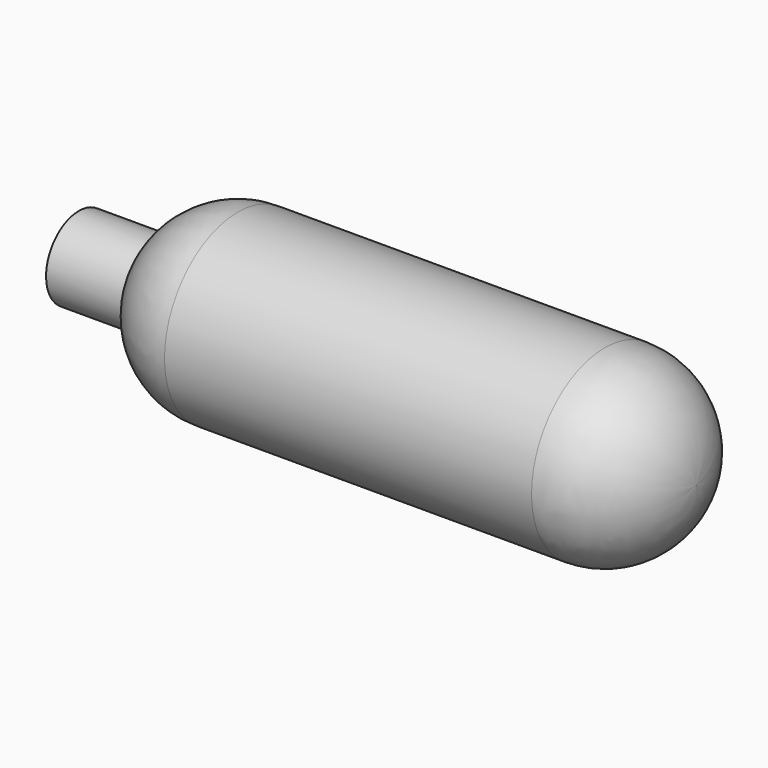
from build123d import *


# Not quite as in the source:
# - a fillet or chamfer that OpenCascade refuses, or shapes differently, is made with other operations: its cross-section is extruded or revolved along the edge and cut away or added


with BuildPart() as f1:
    # F0 (on Front) → F1 (revolve)
    with BuildSketch(Plane.XZ):
        Polygon((0, 4.2418), (0, 0), (64.008, 0), (64.008, 9.4996), (56.007, 9.4996), (36.0045, 9.4996), (16.002, 9.4996), (8.001, 9.4996), (8.001, 4.2418), align=None)
    revolve(axis=Axis((32.004, 0, 0), (1, 0, 0)))

    # F2: fillet of radius 9.4742 on 3 edges, made by hand

    # F2_s1 → F2_t2 (revolve, cut)
    with BuildSketch(Plane.XZ):
        with BuildLine():
            ThreePointArc((54.5338, 9.4996), (61.2330710663, 6.7246710663), (64.008, 0.0254))
            Line((64.008, 0.0254), (64.008, 9.4996))
            Line((64.008, 9.4996), (54.5338, 9.4996))
        make_face()
    revolve(axis=Axis((64.008, 0, 0), (1, 0, 0)), mode=Mode.SUBTRACT)

    # F2_s3 → F2_t4 (revolve, cut)
    with BuildSketch(Plane.XZ):
        with BuildLine():
            ThreePointArc((8.001, 4.2418), (11.4945826612, 8.078582058), (16.4852463826, 9.4996))
            Line((16.4852463826, 9.4996), (8.001, 9.4996))
            Line((8.001, 9.4996), (8.001, 4.2418))
        make_face()
    revolve(axis=Axis((8.001, 0, 0), (1, 0, 0)), mode=Mode.SUBTRACT)


solid = f1.part
